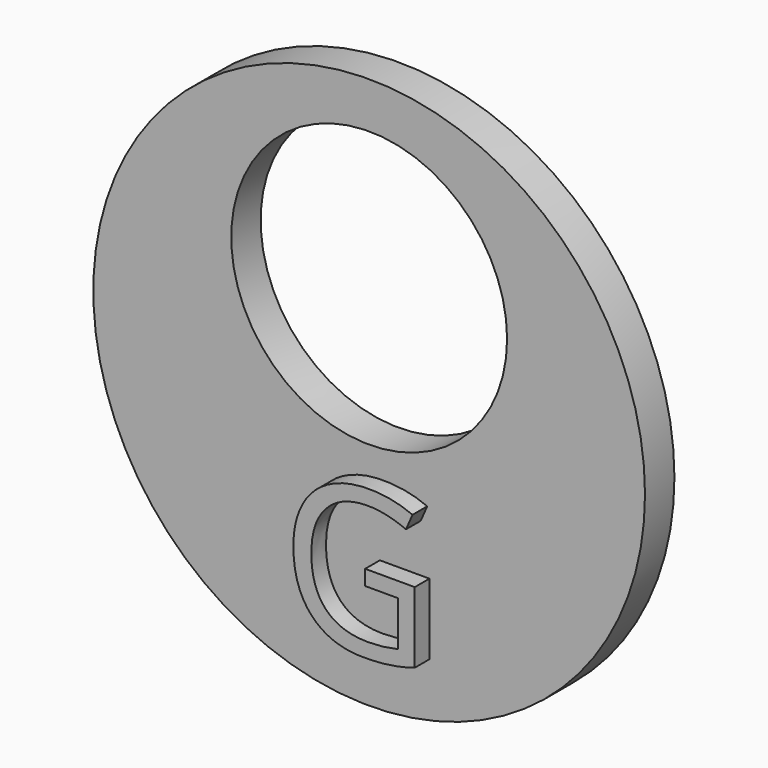
from build123d import *

# Parameters (mm, degrees)
F0_R         = 15
F0_R_2       = 7.5
F1_DEPTH     = 2
F2_TEXT_SIZE = 11.115935736
F3_DEPTH     = 1


# Not quite as in the source:
# - Text() gives the source's letters only with a copy of the font that has no kerning and outlines rounded to 1/6400 em; it was checked with that copy


with BuildPart() as f1:
    # F0 (on Front) → F1 (new body)
    with BuildSketch(Plane.XZ):
        Circle(F0_R)
        with Locations((0, 5)):
            Circle(F0_R_2, mode=Mode.SUBTRACT)
    extrude(amount=F1_DEPTH)

    # F2 (on face) → F3 (join)
    with BuildSketch(Plane.XZ.offset(2)):
        with Locations((-4, -12.0034737299)):
            Text('G', F2_TEXT_SIZE, font='Open Sans', text_align=(TextAlign.LEFT, TextAlign.BOTTOM))
    extrude(amount=F3_DEPTH)


solid = f1.part
